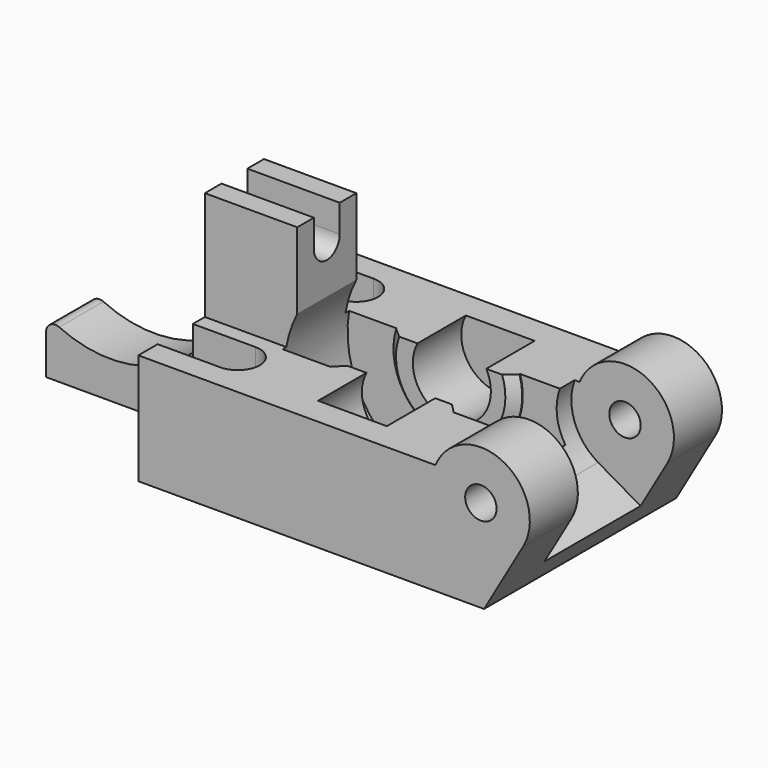
from build123d import *

# Parameters (mm, degrees)
F0_R         = 1.7
F1_DEPTH     = 13
F3_DEPTH     = 12.001
F5_DEPTH     = 6.5
F6_W         = 10
F6_H         = 8
F7_DEPTH     = 11.8
F9_DEPTH     = 42.381
F10_R        = 4.225
F11_DEPTH    = 10
F12_R        = 7.5
F13_DEPTH    = 3.45
F16_R        = 12
F16_R_2      = 6.97
F17_DEPTH    = 4.5
F18_T4_ANGLE = 257.8909092885
F18_T7_ANGLE = 257.8909092885
F20_DEPTH    = 2.9885
F22_DEPTH    = 2


# Not quite as in the source:
# - a fillet or chamfer that OpenCascade refuses, or shapes differently, is made with other operations: its cross-section is extruded or revolved along the edge and cut away or added


with BuildPart() as f1:
    # F0 (on Front) → F1 (new body, symmetric)
    with BuildSketch(Plane.XZ):
        with BuildLine():
            Line((-37.08, 2), (-37.08, -10))
            Line((-37.08, -10), (0.3464101615, -10))
            Line((0.3464101615, -10), (4.5899346401, -2.65))
            ThreePointArc((4.5899346401, -2.65), (2.3304380027, 4.760153224), (-4.9081564767, 2))
            Line((-4.9081564767, 2), (-37.08, 2))
        make_face()
        Circle(F0_R, mode=Mode.SUBTRACT)
    extrude(amount=F1_DEPTH, both=True)

    # F2 (on face) → F3 (cut, through all)
    with BuildSketch(Plane.XY.offset(2)):
        with BuildLine():
            Line((-30.31, 10.385), (-37.08, 10.385))
            Line((-37.08, 10.385), (-37.08, 5.625))
            Line((-37.08, 5.625), (-30.31, 5.625))
            ThreePointArc((-30.31, 5.625), (-27.93, 8.005), (-30.31, 10.385))
        make_face()
        with BuildLine():
            ThreePointArc((-30.31, -10.385), (-27.93, -8.005), (-30.31, -5.625))
            Line((-30.31, -5.625), (-37.08, -5.625))
            Line((-37.08, -5.625), (-37.08, -10.385))
            Line((-37.08, -10.385), (-30.31, -10.385))
        make_face()
    extrude(amount=-F3_DEPTH, mode=Mode.SUBTRACT)

    # F4 (on Front) → F5 (cut, symmetric)
    with BuildSketch(Plane.XZ):
        with BuildLine():
            Line((5.8, -10.0458946839), (5.8, 0))
            ThreePointArc((5.8, 0), (-2.9, 5.0229473419), (-2.9, -5.0229473419))
            Line((-2.9, -5.0229473419), (5.8, -10.0458946839))
        make_face()
    extrude(amount=F5_DEPTH, both=True, mode=Mode.SUBTRACT)

    # F6 (on face) → F7 (join)
    with BuildSketch(Plane.XY.offset(2)):
        with Locations((-32.08, 0)):
            Rectangle(F6_W, F6_H)
    extrude(amount=F7_DEPTH)

    # F8 (on face) → F9 (cut, through all)
    with BuildSketch(Plane(origin=(-37.08, 0, 0), x_dir=(0, -1, 0), z_dir=(-1, 0, 0))):
        with BuildLine():
            Line((1.75, 13.8), (-1.75, 13.8))
            Line((-1.75, 13.8), (-1.75, 10.8))
            ThreePointArc((-1.75, 10.8), (0, 9.05), (1.75, 10.8))
            Line((1.75, 10.8), (1.75, 13.8))
        make_face()
    extrude(amount=-F9_DEPTH, mode=Mode.SUBTRACT)

    # F10 (on Front) → F11 (cut, symmetric)
    with BuildSketch(Plane.XZ):
        with Locations((-16.3, 0)):
            Circle(F10_R)
    extrude(amount=F11_DEPTH, both=True, mode=Mode.SUBTRACT)

    # F12 (on Front) → F13 (cut, symmetric)
    with BuildSketch(Plane.XZ):
        with Locations((-16.3, 0)):
            Circle(F12_R)
    extrude(amount=F13_DEPTH, both=True, mode=Mode.SUBTRACT)

    # F16 (on Front) → F17 (cut, symmetric)
    with BuildSketch(Plane.XZ):
        with Locations((-16.4292231202, 0)):
            Circle(F16_R)
        with Locations((-16.4292231202, 0)):
            Circle(F16_R_2, mode=Mode.SUBTRACT)
    extrude(amount=F17_DEPTH, both=True, mode=Mode.SUBTRACT)

    # F18: chamfer of 1.05 x 0.9699305265 on 2 edges, made by hand


with BuildPart() as f18_tool2:
    # F18_s3 → F18_t4 (revolve)
    with BuildSketch(Plane(origin=(-6.4914021144, 0, -8.0318361717), x_dir=(0, 1, 0), z_dir=(0.6285802661, 0, 0.7777447197))):
        Polygon((-3.45, 18.7778110045), (-4.5, 19.747741531), (-3.45, 19.747741531), align=None)
    revolve(axis=Axis((-16.4292231202, -3.45, 0), (0, -1, 0)), revolution_arc=F18_T4_ANGLE)

    split(bisect_by=Plane.XZ.offset(4.5), keep=Keep.BOTTOM)


with BuildPart() as f1_1:
    add(f1.part)

    # F18_t1: cut F18_tool2
    add(f18_tool2.part, mode=Mode.SUBTRACT)

    # F18_s6 → F18_t7 (revolve, cut)
    with BuildSketch(Plane(origin=(-6.4914021144, 0, 8.0318361717), x_dir=(0, 1, 0), z_dir=(-0.6285802661, 0, 0.7777447197))):
        Polygon((4.4199305265, 5.807741531), (3.45, 6.857741531), (3.45, 5.807741531), align=None)
    revolve(axis=Axis((-16.4292231202, 3.45, 0), (0, 1, 0)), revolution_arc=F18_T7_ANGLE, mode=Mode.SUBTRACT)

    # F19 (on Front) → F20 (join, symmetric)
    with BuildSketch(Plane.XZ):
        with BuildLine():
            Line((-37.08, -10), (-37.08, 0))
            ThreePointArc((-37.08, 0), (-44.4762536163, -5.4872309342), (-53.6579068221, -4.7720279633))
            ThreePointArc((-53.6579068221, -4.7720279633), (-54.617543869, -4.8353446309), (-55.08, -5.6785804158))
            Line((-55.08, -5.6785804158), (-55.08, -10))
            Line((-55.08, -10), (-37.08, -10))
        make_face()
    extrude(amount=F20_DEPTH, both=True)

    # F21 (on face) → F22 (cut)
    with BuildSketch(Plane(origin=(0, -6.5, 0), x_dir=(-1, 0, 0), z_dir=(0, 1, 0))):
        Polygon((-3.579571669, 0), (-1.7897858345, -3.1), (1.7897858345, -3.1), (3.579571669, 0), (1.7897858345, 3.1), (-1.7897858345, 3.1), align=None)
    extrude(amount=-F22_DEPTH, mode=Mode.SUBTRACT)


solid = f1_1.part
